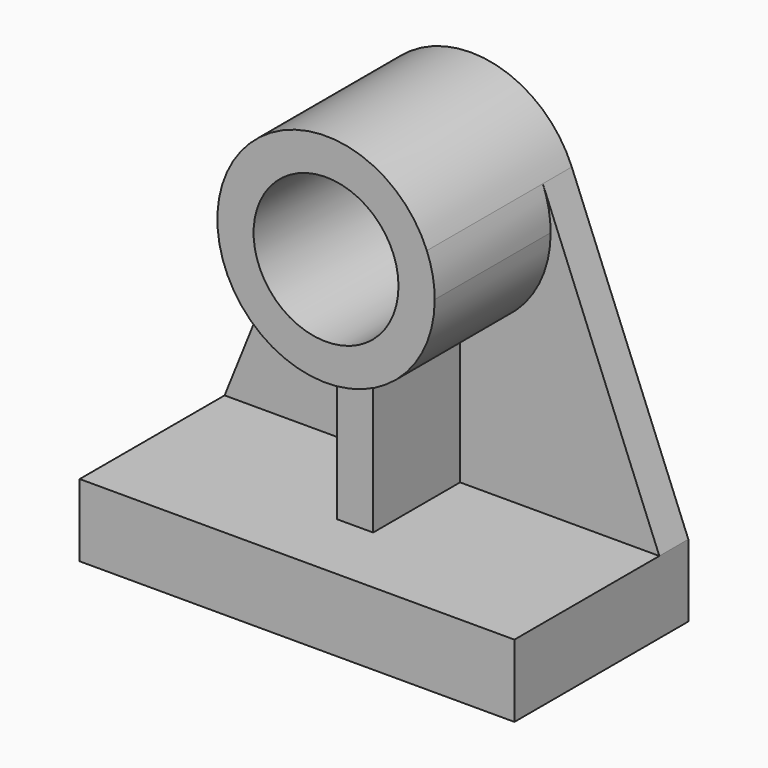
from build123d import *

# Parameters (mm, degrees)
F1_DEPTH      = 25.4
F2_W          = 304.8
F2_H          = 50.8
F3_DEPTH      = 127
F5_R          = 50.8
F6_DEPTH      = 25.401
F7_DEPTH      = 101.6
F8_DEPTH      = 127.001
F8_DEPTH_BACK = 25.401
F10_DEPTH     = 76.2


with BuildPart() as f1:
    # F0 (on Front) → F1 (new body)
    with BuildSketch(Plane.XZ):
        with BuildLine():
            Line((0, 50.8), (0, 0))
            Line((0, 0), (304.8, 0))
            Line((304.8, 0), (304.8, 50.8))
            Line((304.8, 50.8), (223.0993426351, 254))
            ThreePointArc((223.0993426351, 254), (152.4, 301.7739036981), (81.7006573649, 254))
            Line((81.7006573649, 254), (0, 50.8))
        make_face()
    extrude(amount=F1_DEPTH)

    # F2 (on face) → F3 (join)
    with BuildSketch(Plane.XZ.offset(25.4)):
        with Locations((152.4, 25.4)):
            Rectangle(F2_W, F2_H)
    extrude(amount=F3_DEPTH)

    # F5 (on face) → F6 (cut, through all)
    with BuildSketch(Plane.XZ.offset(25.4)):
        with Locations((152.4, 225.5739036981)):
            Circle(F5_R)
    extrude(amount=-F6_DEPTH, mode=Mode.SUBTRACT)

    # F4 (on face) → F7 (join)
    with BuildSketch(Plane.XZ.offset(25.4)):
        with BuildLine():
            ThreePointArc((81.7006573649, 254), (137.9232929986, 150.7617057996), (228.6, 225.5739036981))
            ThreePointArc((228.6, 225.5739036981), (227.2121978984, 240.0506106994), (223.0993426351, 254))
            ThreePointArc((223.0993426351, 254), (152.4, 301.7739036981), (81.7006573649, 254))
        make_face()
    extrude(amount=F7_DEPTH)

    # F5 (on face) → F8 (cut, two sides)
    with BuildSketch(Plane.XZ.offset(25.4)) as f8_sk:
        with Locations((152.4, 225.5739036981)):
            Circle(F5_R)
    extrude(amount=F8_DEPTH, mode=Mode.SUBTRACT)
    extrude(f8_sk.sketch, amount=-F8_DEPTH_BACK, mode=Mode.SUBTRACT)

    # F9 (on face) → F10 (join)
    with BuildSketch(Plane.XZ.offset(25.4)):
        with BuildLine():
            Line((139.7, 150.4396904527), (139.7, 50.8))
            Line((139.7, 50.8), (165.1, 50.8))
            Line((165.1, 50.8), (165.1, 150.4396904527))
            ThreePointArc((165.1, 150.4396904527), (152.4, 149.3739036981), (139.7, 150.4396904527))
        make_face()
    extrude(amount=F10_DEPTH)


solid = f1.part
